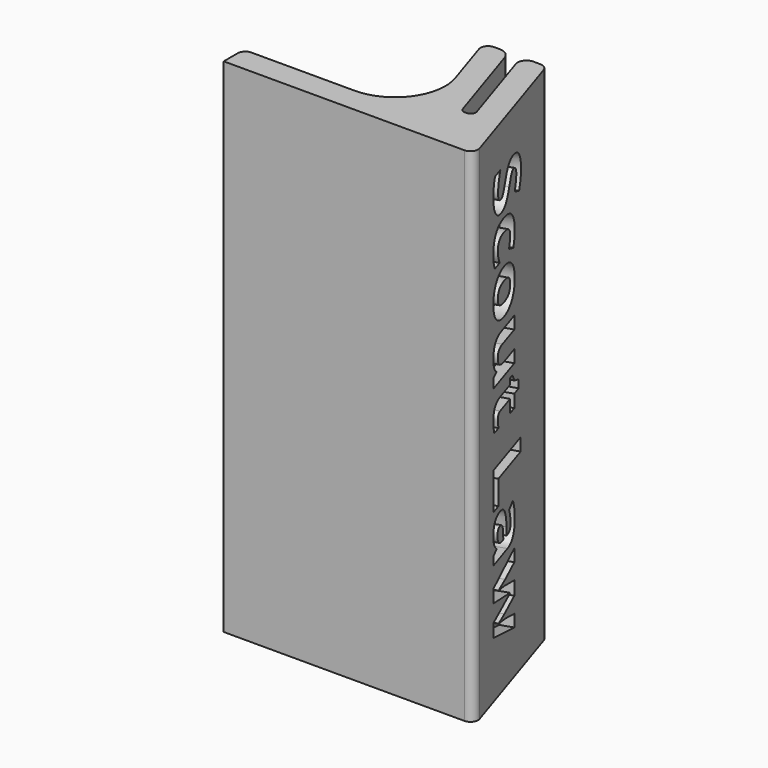
from build123d import *

# Parameters (mm, degrees)
F1_DEPTH     = 40
F2_TEXT_SIZE = 6.6465072238
F3_DEPTH     = 1


# Not quite as in the source:
# - Text() gives the source's letters only with a copy of the font that has no kerning and outlines rounded to 1/6400 em; it was checked with that copy


with BuildPart() as f1:
    # F0 (on Top) → F1 (new body)
    with BuildSketch(Plane.XY):
        with BuildLine():
            Line((-34.1906128108, 7.3942965377), (-15.0164419631, 7.3942965377))
            ThreePointArc((-15.0164419631, 7.3942965377), (-14.5310317665, 7.6416253863), (-14.4458080533, 8.1797067343))
            Line((-14.4458080533, 8.1797067343), (-17.9324893738, 18.9106084338))
            ThreePointArc((-17.9324893738, 18.9106084338), (-18.1867792586, 19.2606084338), (-18.5982289352, 19.3942965377))
            Line((-18.5982289352, 19.3942965377), (-19.1261818213, 19.3942965377))
            ThreePointArc((-19.1261818213, 19.3942965377), (-19.6924937174, 19.1057462143), (-19.7919213827, 18.4779846416))
            Line((-19.7919213827, 18.4779846416), (-17.6604217574, 11.9179033355))
            ThreePointArc((-17.6604217574, 11.9179033355), (-17.7172375662, 11.5591824368), (-18.0408443639, 11.3942965377))
            Line((-18.0408443639, 11.3942965377), (-18.1996745846, 11.3942965377))
            ThreePointArc((-18.1996745846, 11.3942965377), (-18.4347886855, 11.47068974), (-18.5800971911, 11.67068974))
            Line((-18.5800971911, 11.67068974), (-20.8651351773, 18.7033135321))
            ThreePointArc((-20.8651351773, 18.7033135321), (-21.2284064413, 19.2033135321), (-21.8161916936, 19.3942965377))
            Line((-21.8161916936, 19.3942965377), (-22.2638200133, 19.3942965377))
            ThreePointArc((-22.2638200133, 19.3942965377), (-22.74923021, 19.1469676891), (-22.8344539231, 18.6088863411))
            Line((-22.8344539231, 18.6088863411), (-21.54175382, 14.6303645152))
            ThreePointArc((-21.54175382, 14.6303645152), (-22.1099119077, 11.0431555285), (-25.3459798852, 9.3942965377))
            Line((-25.3459798852, 9.3942965377), (-33.5906128108, 9.3942965377))
            ThreePointArc((-33.5906128108, 9.3942965377), (-34.0148768795, 9.2185606064), (-34.1906128108, 8.7942965377))
            Line((-34.1906128108, 8.7942965377), (-34.1906128108, 7.3942965377))
        make_face()
    extrude(amount=F1_DEPTH)

    # F2 (on face) → F3 (cut)
    with BuildSketch(Plane(origin=(-10.6624006397, -3.464423977, 0), x_dir=(-0.3090169944, 0.9510565163, 0), z_dir=(0.9510565163, 0.3090169944, 0))):
        with Locations(Location((14.7410161449, 37), (0, 0, -90))):
            Text('Scout Law', F2_TEXT_SIZE, font='Open Sans', font_style=FontStyle.BOLD, text_align=(TextAlign.LEFT, TextAlign.BOTTOM))
    extrude(amount=-F3_DEPTH, mode=Mode.SUBTRACT)


solid = f1.part
